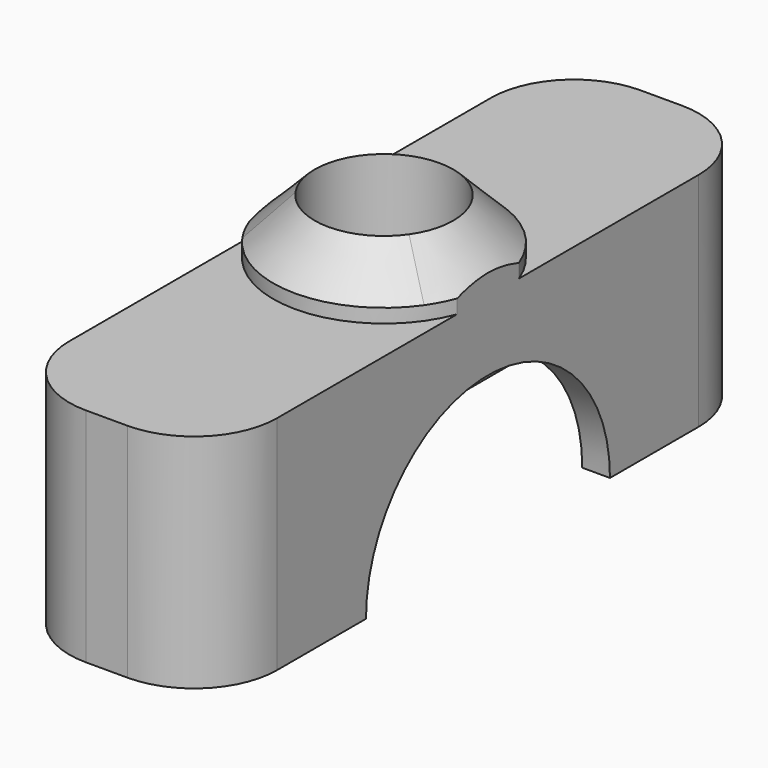
from build123d import *

# Parameters (mm, degrees)
F0_W         = 15
F0_H         = 50
F1_DEPTH     = 16
F3_DEPTH     = 25
F4_T         = -2
F5_R         = 6
F6_R         = 5
F7_DEPTH     = 25
F9_DEPTH     = 4
F10_R        = 5
F11_DEPTH    = 25
F12_T2_ANGLE = 249.8880129875
F12_T4_ANGLE = 220.6883825687
F13_R        = 2
F13_R_2      = 1.25
F14_DEPTH    = 14


# Not quite as in the source:
# - a fillet or chamfer that OpenCascade refuses, or shapes differently, is made with other operations: its cross-section is extruded or revolved along the edge and cut away or added


with BuildPart() as f1:
    # F0 (on Top) → F1 (new body)
    with BuildSketch(Plane.XY):
        with Locations((-7.5, 25)):
            Rectangle(F0_W, F0_H)
    extrude(amount=F1_DEPTH)

    # F2 (on face) → F3 (cut)
    with BuildSketch(Plane.YZ):
        with BuildLine():
            Line((14, 0), (36, 0))
            ThreePointArc((36, 0), (25, 11), (14, 0))
        make_face()
    extrude(amount=-F3_DEPTH, mode=Mode.SUBTRACT)

    # F4
    f4_openings = [f1.faces().sort_by_distance(p)[0] for p in [
        (-7.5, 25, 11),
        (-7.5, 7, 0),
        (-7.5, 43, 0),
    ]]
    offset(amount=F4_T, openings=f4_openings)

    # F5
    f5_edges = [f1.edges().sort_by_distance(p)[0] for p in [
        (0, 0, 8),
        (0, 50, 8),
        (-15, 50, 8),
        (-15, 0, 8),
    ]]
    fillet(f5_edges, radius=F5_R)

    # F6 (on face) → F7 (cut)
    with BuildSketch(Plane.XY.offset(16)):
        with Locations((-7.5, 25)):
            Circle(F6_R)
    extrude(amount=-F7_DEPTH, mode=Mode.SUBTRACT)

    # F8 (on face) → F9 (join)
    with BuildSketch(Plane.XY.offset(16)):
        with BuildLine():
            ThreePointArc((0, 27.7838821814), (-7.5, 33), (-15, 27.7838821814))
            Line((-15, 27.7838821814), (-15, 22.2161178186))
            ThreePointArc((-15, 22.2161178186), (-7.5, 17), (0, 22.2161178186))
            Line((0, 22.2161178186), (0, 27.7838821814))
        make_face()
    extrude(amount=F9_DEPTH)

    # F10 (on face) → F11 (cut)
    with BuildSketch(Plane.XY.offset(20)):
        with Locations((-7.5, 25)):
            Circle(F10_R)
    extrude(amount=-F11_DEPTH, mode=Mode.SUBTRACT)

    # F12: chamfer of 3 on 4 edges, made by hand

    # F12_s1 → F12_t2 (revolve, cut)
    with BuildSketch(Plane(origin=(9.2772397602, 13.2768682197, 0), x_dir=(0, 0, 1), z_dir=(-0.572775629, -0.8197121927, 0))):
        Polygon((20, 15.4672321702), (17, 12.4672321702), (20, 12.4672321702), align=None)
    revolve(axis=Axis((-7.5, 25, 20), (0, 0, 1)), revolution_arc=F12_T2_ANGLE, mode=Mode.SUBTRACT)

    # F12_s3 → F12_t4 (revolve, cut)
    with BuildSketch(Plane(origin=(7.2428078971, 19.5335392611, 0), x_dir=(0, 0, 1), z_dir=(0.3476589265, 0.93762107, 0))):
        Polygon((17, -23.7236311869), (20, -20.7236311869), (20, -23.7236311869), align=None)
    revolve(axis=Axis((-7.5, 25, 20), (0, 0, 1)), revolution_arc=F12_T4_ANGLE, mode=Mode.SUBTRACT)

    # F13 (on face) → F14 (join)
    with BuildSketch(Plane(origin=(0, 0, 14), x_dir=(1, 0, 0), z_dir=(0, 0, -1))):
        with Locations((-7.5, -3)):
            Circle(F13_R)
        with Locations((-7.5, -3)):
            Circle(F13_R_2, mode=Mode.SUBTRACT)
        with Locations((-7.5, -47)):
            Circle(F13_R)
        with Locations((-7.5, -47)):
            Circle(F13_R_2, mode=Mode.SUBTRACT)
    extrude(amount=F14_DEPTH)


solid = f1.part
